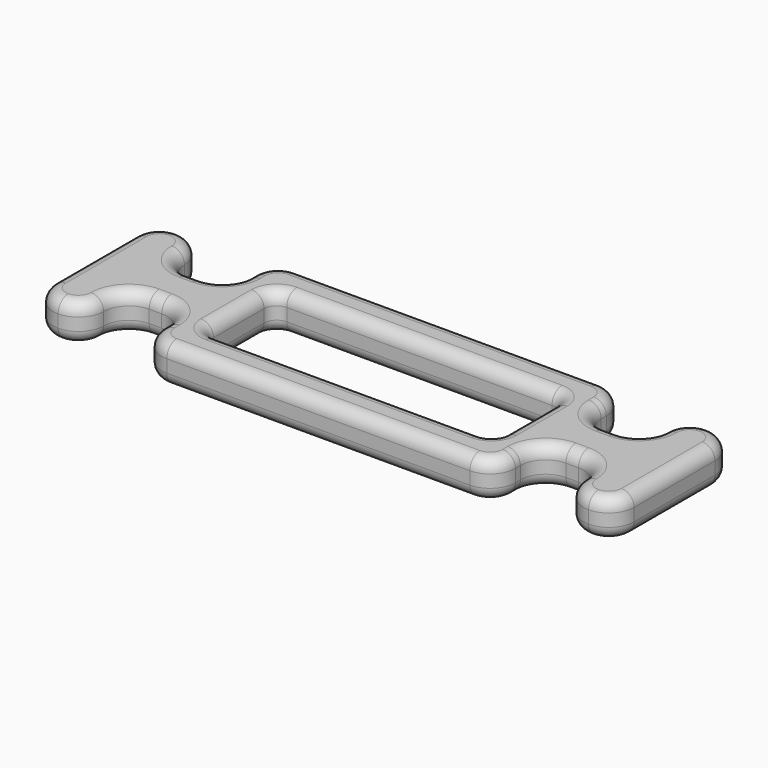
from build123d import *

# Parameters (mm, degrees)
F0_W     = 23
F0_H     = 7
F1_DEPTH = 3
F2_R     = 1.99999
F3_R     = 1


# Not quite as in the source:
# - a fillet or chamfer is up to 0.001 mm smaller than in the source, because OpenCascade refuses the exact size
# - a feature names something its author has since deleted; it is built from what else it names


with BuildPart() as f1:
    # F0 (on Top) → F1 (new body)
    with BuildSketch(Plane.XY):
        Polygon((14, 6.5), (-14, 6.5), (-14, 2), (-19, 2), (-19, 6), (-23, 6), (-23, 0), (-23, -6), (-19, -6), (-19, -2), (-14, -2), (-14, -6.5), (14, -6.5), (14, -2), (19, -2), (19, -6), (23, -6), (23, 0), (23, 6), (19, 6), (19, 2), (14, 2), align=None)
        Rectangle(F0_W, F0_H, mode=Mode.SUBTRACT)
    extrude(amount=F1_DEPTH)

    # F2 (radius 2 in the source; OpenCascade refuses exactly that, so slightly less here)
    f2_edges = [f1.edges().sort_by_distance(p)[0] for p in [
        (14, 6.5, 1.5),
        (-14, 6.5, 1.5),
        (14, -2, 1.5),
        (-14, -2, 1.5),
        (19, -2, 1.5),
        (19, 2, 1.5),
        (-19, 2, 1.5),
        (-19, -2, 1.5),
        (-19, -6, 1.5),
        (-23, -6, 1.5),
        (-23, 6, 1.5),
        (19, -6, 1.5),
        (23, -6, 1.5),
        (-19, 6, 1.5),
        (19, 6, 1.5),
        (23, 6, 1.5),
        (14, 2, 1.5),
        (14, -6.5, 1.5),
        (-14, -6.5, 1.5),
        (-14, 2, 1.5),
    ]]
    fillet(f2_edges, radius=F2_R)

    # F3
    f3_edges = [f1.edges().sort_by_distance(p)[0] for p in [
        (-11.5, 3.5, 1.5),
        (-11.5, -3.5, 1.5),
        (0, 6.5, 0),
        (13.414216, 5.914216, 0),
        (-13.414216, 5.914216, 0),
        (14, 4.25, 0),
        (-14, 4.25, 0),
        (14.585784, 2.585784, 0),
        (-14.585784, 2.585784, 0),
        (16.5, 2, 0),
        (-16.5, 2, 0),
        (18.414216, 2.585784, 0),
        (-18.414216, 2.585784, 0),
        (19, 4, 0),
        (-19, 4, 0),
        (19.585784, 5.414216, 0),
        (-19.585784, 5.414216, 0),
        (21, 6, 0),
        (-21, 6, 0),
        (22.414216, 5.414216, 0),
        (-22.414216, 5.414216, 0),
        (23, 0, 0),
        (-23, 0, 0),
        (22.414216, -5.414216, 0),
        (-22.414216, -5.414216, 0),
        (21, -6, 0),
        (-21, -6, 0),
        (19.585784, -5.414216, 0),
        (-19.585784, -5.414216, 0),
        (19, -4, 0),
        (-19, -4, 0),
        (18.414216, -2.585784, 0),
        (-18.414216, -2.585784, 0),
        (16.5, -2, 0),
        (-16.5, -2, 0),
        (14.585784, -2.585784, 0),
        (-14.585784, -2.585784, 0),
        (14, -4.25, 0),
        (-14, -4.25, 0),
        (13.414216, -5.914216, 0),
        (-13.414216, -5.914216, 0),
        (0, -6.5, 0),
        (0, 3.5, 0),
        (11.5, 0, 0),
        (0, -3.5, 0),
        (-11.5, 0, 0),
        (0, 6.5, 3),
        (13.414216, 5.914216, 3),
        (-13.414216, 5.914216, 3),
        (14, 4.25, 3),
        (-14, 4.25, 3),
        (14.585784, 2.585784, 3),
        (-14.585784, 2.585784, 3),
        (16.5, 2, 3),
        (-16.5, 2, 3),
        (18.414216, 2.585784, 3),
        (-18.414216, 2.585784, 3),
        (19, 4, 3),
        (-19, 4, 3),
        (19.585784, 5.414216, 3),
        (-19.585784, 5.414216, 3),
        (21, 6, 3),
        (-21, 6, 3),
        (22.414216, 5.414216, 3),
        (-22.414216, 5.414216, 3),
        (23, 0, 3),
        (-23, 0, 3),
        (22.414216, -5.414216, 3),
        (-22.414216, -5.414216, 3),
        (21, -6, 3),
        (-21, -6, 3),
        (19.585784, -5.414216, 3),
        (-19.585784, -5.414216, 3),
        (19, -4, 3),
        (-19, -4, 3),
        (18.414216, -2.585784, 3),
        (-18.414216, -2.585784, 3),
        (16.5, -2, 3),
        (-16.5, -2, 3),
        (14.585784, -2.585784, 3),
        (-14.585784, -2.585784, 3),
        (14, -4.25, 3),
        (-14, -4.25, 3),
        (13.414216, -5.914216, 3),
        (-13.414216, -5.914216, 3),
        (0, -6.5, 3),
        (0, 3.5, 3),
        (11.5, 0, 3),
        (0, -3.5, 3),
        (-11.5, 0, 3),
        (11.5, 3.5, 1.5),
        (11.5, -3.5, 1.5),
    ]]
    fillet(f3_edges, radius=F3_R)


solid = f1.part
